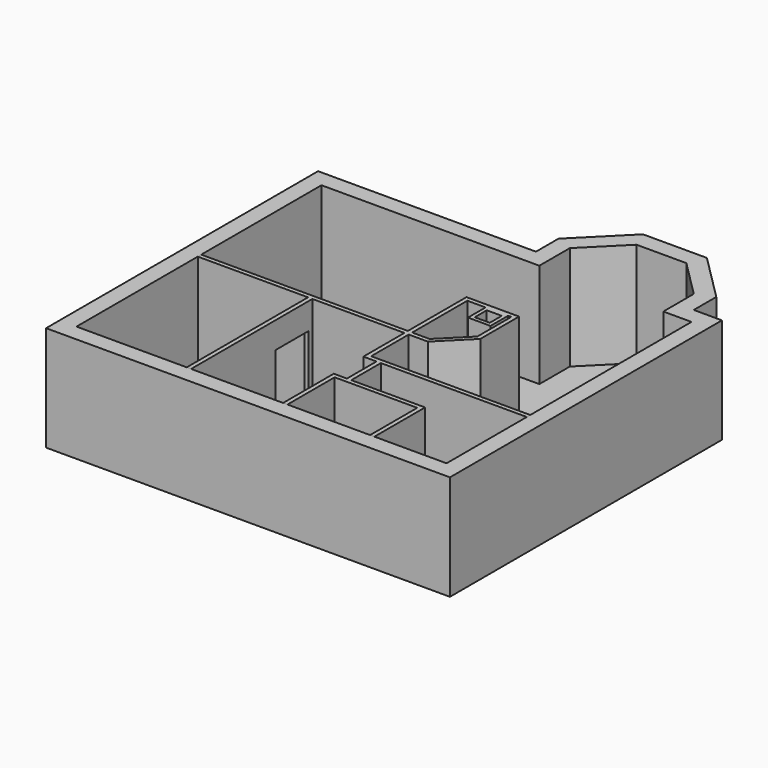
from build123d import *

# Parameters (mm, degrees)
F0_W     = 2935
F0_H     = 4035
F0_W_2   = 400
F0_H_2   = 400
F0_W_3   = 2200
F0_H_3   = 1570
F1_DEPTH = 25
F2_DEPTH = 2800
F3_DEPTH = 2800
F4_W     = 1100
F4_H     = 2100
F5_DEPTH = 115


with BuildPart() as f1:
    # F0 (on Top) → F1 (new body)
    with BuildSketch(Plane.XY):
        Polygon((-5375, -4525), (5375, -4525), (5375, 4525), (4625, 4525), (4625, 5275), (3375, 6525), (2956.3961030679, 6525), (2086.3961030679, 6525), (1675, 6525), (425, 5275), (425, 4525), (-149.870057106, 4525), (-1879.870057106, 4525), (-2737.3004150391, 4525), (-4467.3004150391, 4525), (-5375, 4525), align=None)
        Polygon((-149.870057106, 4075), (875, 4075), (875, 5088.6038969321), (1861.3961030679, 6075), (2086.3961030679, 6075), (2956.3961030679, 6075), (3188.6038969321, 6075), (4175, 5088.6038969321), (4175, 4075), (4925, 4075), (4925, 2025), (4925, -1290), (4925, -1405), (4925, -4075), (3005, -4075), (2890, -4075), (690, -4075), (575, -4075), (-1875, -4075), (-1990, -4075), (-4925, -4075), (-4925, -40), (-4925, 75), (-4925, 4075), (-4467.3004150391, 4075), (-2737.3004150391, 4075), (-1879.870057106, 4075), align=None, mode=Mode.SUBTRACT)
        Polygon((875, 5088.6038969321), (875, 4075), (-149.870057106, 4075), (-1879.870057106, 4075), (-2737.3004150391, 4075), (-4467.3004150391, 4075), (-4925, 4075), (-4925, 75), (-1875, 75), (575, 75), (575, 2025), (1975, 2025), (4925, 2025), (4925, 4075), (4175, 4075), (4175, 5088.6038969321), (3188.6038969321, 6075), (2956.3961030679, 6075), (2086.3961030679, 6075), (1861.3961030679, 6075), align=None)
        with Locations((-3457.5, -2057.5)):
            Rectangle(F0_W, F0_H)
        Polygon((4925, -1290), (4925, 2025), (1975, 2025), (1975, 734.4722215136), (1200.5277784864, -40), (690, -40), (690, -1290), align=None)
        Polygon((-1875, -775), (-1875, -4075), (575, -4075), (575, -2390), (925, -2390), (925, -1405), (575, -1405), (575, -1290), (575, -40), (-1875, -40), align=None)
        Polygon((4925, -4075), (4925, -1405), (1040, -1405), (1040, -2390), (3005, -2390), (3005, -4075), align=None)
        Polygon((-1875, 75), (-4925, 75), (-4925, -40), (-1990, -40), (-1990, -4075), (-1875, -4075), (-1875, -775), (-1875, -40), (575, -40), (575, -1290), (575, -1405), (925, -1405), (925, -2390), (575, -2390), (575, -4075), (690, -4075), (690, -2505), (2890, -2505), (2890, -4075), (3005, -4075), (3005, -2390), (1040, -2390), (1040, -1405), (4925, -1405), (4925, -1290), (690, -1290), (690, -40), (1200.5277784864, -40), (1975, 734.4722215136), (1975, 2025), (575, 2025), (575, 75), align=None)
        Polygon((1152.8932188135, 75), (690, 75), (690, 1910), (1175, 1910), (1175, 1325), (1775, 1325), (1775, 1910), (1860, 1910), (1860, 782.1067811865), align=None, mode=Mode.SUBTRACT)
        with Locations((1475, 1625)):
            Rectangle(F0_W_2, F0_H_2, mode=Mode.SUBTRACT)
        with Locations((1790, -3290)):
            Rectangle(F0_W_3, F0_H_3)
        Polygon((690, 1910), (690, 75), (1152.8932188135, 75), (1860, 782.1067811865), (1860, 1910), (1775, 1910), (1775, 1325), (1175, 1325), (1175, 1910), align=None)
        with Locations((1475, 1625)):
            Rectangle(F0_W_2, F0_H_2)
    extrude(amount=F1_DEPTH)


with BuildPart() as f2:
    # F0 (on Top) → F2 (new body)
    with BuildSketch(Plane.XY):
        Polygon((-5375, -4525), (5375, -4525), (5375, 4525), (4625, 4525), (4625, 5275), (3375, 6525), (2956.3961030679, 6525), (2086.3961030679, 6525), (1675, 6525), (425, 5275), (425, 4525), (-149.870057106, 4525), (-1879.870057106, 4525), (-2737.3004150391, 4525), (-4467.3004150391, 4525), (-5375, 4525), align=None)
        Polygon((-149.870057106, 4075), (875, 4075), (875, 5088.6038969321), (1861.3961030679, 6075), (2086.3961030679, 6075), (2956.3961030679, 6075), (3188.6038969321, 6075), (4175, 5088.6038969321), (4175, 4075), (4925, 4075), (4925, 2025), (4925, -1290), (4925, -1405), (4925, -4075), (3005, -4075), (2890, -4075), (690, -4075), (575, -4075), (-1875, -4075), (-1990, -4075), (-4925, -4075), (-4925, -40), (-4925, 75), (-4925, 4075), (-4467.3004150391, 4075), (-2737.3004150391, 4075), (-1879.870057106, 4075), align=None, mode=Mode.SUBTRACT)
    extrude(amount=F2_DEPTH)


with BuildPart() as f3:
    # F0 (on Top) → F3 (new body, through all)
    with BuildSketch(Plane.XY):
        Polygon((-1875, 75), (-4925, 75), (-4925, -40), (-1990, -40), (-1990, -4075), (-1875, -4075), (-1875, -775), (-1875, -40), (575, -40), (575, -1290), (575, -1405), (925, -1405), (925, -2390), (575, -2390), (575, -4075), (690, -4075), (690, -2505), (2890, -2505), (2890, -4075), (3005, -4075), (3005, -2390), (1040, -2390), (1040, -1405), (4925, -1405), (4925, -1290), (690, -1290), (690, -40), (1200.5277784864, -40), (1975, 734.4722215136), (1975, 2025), (575, 2025), (575, 75), align=None)
        Polygon((1152.8932188135, 75), (690, 75), (690, 1910), (1175, 1910), (1175, 1325), (1775, 1325), (1775, 1910), (1860, 1910), (1860, 782.1067811865), align=None, mode=Mode.SUBTRACT)
        with Locations((1475, 1625)):
            Rectangle(F0_W_2, F0_H_2, mode=Mode.SUBTRACT)
    extrude(amount=F3_DEPTH)

    # F4 (on face) → F5 (cut, through all)
    with BuildSketch(Plane(origin=(-1990, 0, 0), x_dir=(0, -1, 0), z_dir=(-1, 0, 0))):
        with Locations((715, 1050)):
            Rectangle(F4_W, F4_H)
    extrude(amount=-F5_DEPTH, mode=Mode.SUBTRACT)


solid = Compound([f1.part, f2.part, f3.part])
